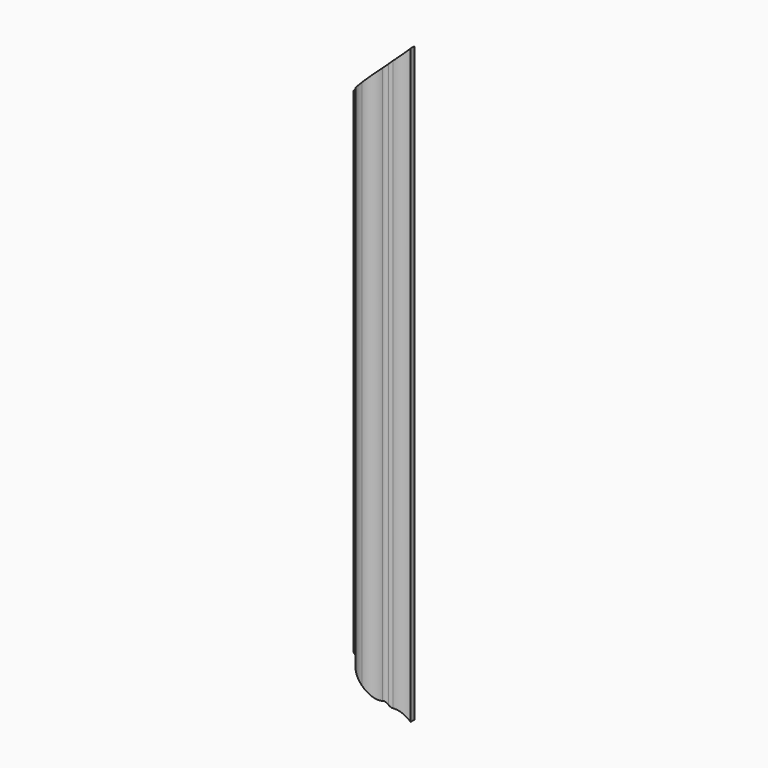
from build123d import *

# Parameters (mm, degrees)
F1_DEPTH = 381
F2_R     = 2.54
F3_R     = 2.54
F4_R     = 2.54
F5_W     = 6.35
F5_H     = 381
F6_DEPTH = 7.62
F8_DEPTH = 17.4635001


# Not quite as in the source:
# - ends of sketch curves that miss each other by under 0.0002 mm in the source are joined


with BuildPart() as f1:
    # F0 (on Top) → F1 (new body)
    with BuildSketch(Plane.XY):
        with BuildLine():
            Line((15.875, 5.55625), (15.875, 8.73125))
            Line((15.875, 8.73125), (-15.875, 8.73125))
            Line((-15.875, 8.73125), (-15.875, -0.79375))
            Line((-15.875, -0.79375), (-12.7, -0.79375))
            ThreePointArc((-12.7, -0.79375), (-9.8710707302, -6.4481459867), (-3.9751, -8.73125))
            Line((-3.9751, -8.73125), (-3.96875, -8.73125))
            ThreePointArc((-3.96875, -8.73125), (1.9312218072, -6.4502821485), (4.7625, -0.79375))
            Line((4.7625, -0.79375), (7.9375, -0.79375))
            ThreePointArc((7.9375, -0.79375), (10.9883747468, 3.5285940665), (15.875, 5.55625))
        make_face()
    extrude(amount=F1_DEPTH)

    # F2
    f2_edges = [f1.edges().sort_by_distance(p)[0] for p in [
        (7.9375, -0.79375, 190.5),
    ]]
    fillet(f2_edges, radius=F2_R)

    # F3
    f3_edges = [f1.edges().sort_by_distance(p)[0] for p in [
        (-12.7, -0.79375, 190.5),
    ]]
    fillet(f3_edges, radius=F3_R)

    # F4
    f4_edges = [f1.edges().sort_by_distance(p)[0] for p in [
        (4.7625, -0.79375, 190.5),
    ]]
    fillet(f4_edges, radius=F4_R)

    # F5 (on face) → F6 (cut)
    with BuildSketch(Plane(origin=(0, 8.73125, 0), x_dir=(-1, 0, 0), z_dir=(0, 1, 0))):
        with Locations((12.7, 190.5)):
            Rectangle(F5_W, F5_H)
    extrude(amount=-F6_DEPTH, mode=Mode.SUBTRACT)

    # F7 (on face) → F8 (cut, through all)
    with BuildSketch(Plane(origin=(0, 8.73125, 0), x_dir=(-1, 0, 0), z_dir=(0, 1, 0))):
        Polygon((15.875, 0), (15.875, 31.75), (-15.875, 0), align=None)
        Polygon((15.875, 381), (-15.875, 381), (15.875, 349.25), align=None)
    extrude(amount=-F8_DEPTH, mode=Mode.SUBTRACT)


solid = f1.part
